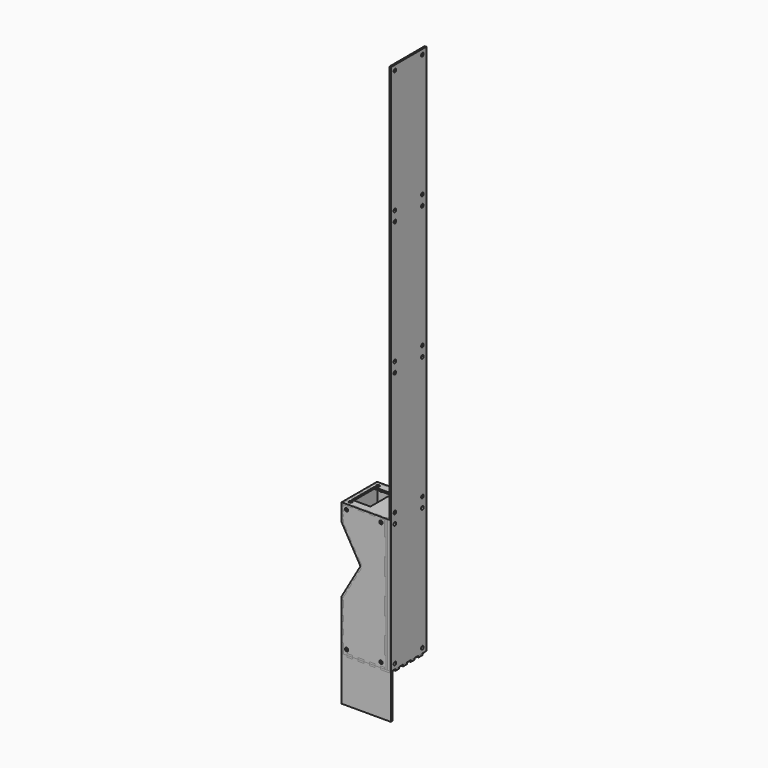
from build123d import *

# Parameters (mm, degrees)
F5_W      = 7
F5_H      = 3
F5_W_2    = 10
F5_W_3    = 3
F5_H_2    = 5.9052353799
F5_H_3    = 8.75
F5_R      = 3
F5_W_4    = 33.25
F5_H_4    = 50
F5_H_5    = 6.8447646201
F27_DEPTH = 3
F7_R      = 3
F7_W      = 3
F7_H      = 30
F7_H_2    = 31.25
F7_H_3    = 22.5
F28_DEPTH = 3
F3_R      = 3
F29_DEPTH = 3
F9_W      = 7
F9_H      = 3
F9_W_2    = 10
F9_R      = 3
F9_W_3    = 3
F9_H_2    = 15.5947646201
F9_H_3    = 8.75
F9_H_4    = 5.9052353799
F30_DEPTH = 3
F11_R     = 3
F31_DEPTH = 3
F32_DEPTH = 3
F33_DEPTH = 3
F34_DEPTH = 3
F35_DEPTH = 3
F36_DEPTH = 3
F37_DEPTH = 3
F38_DEPTH = 3
F39_DEPTH = 3
F40_DEPTH = 3
F19_R     = 25
F41_DEPTH = 3
F42_DEPTH = 3
F21_R     = 3
F43_DEPTH = 3
F22_W     = 80
F22_H     = 240
F22_R     = 3
F22_W_2   = 2
F22_H_2   = 144
F22_W_3   = 12
F44_DEPTH = 3
F24_W     = 80
F24_H     = 240
F24_R     = 3
F45_DEPTH = 3
F26_R     = 3
F26_W     = 3
F26_H     = 2
F26_W_2   = 33.25
F26_H_2   = 50
F46_DEPTH = 3
F47_DEPTH = 3
F25_W     = 7
F25_H     = 3
F25_W_2   = 3
F25_H_2   = 8.75
F25_W_3   = 10
F25_H_3   = 5.9052353799
F48_DEPTH = 3
F25_H_4   = 6.8447646201
F49_DEPTH = 3


# Not quite as in the source:
# - a feature names something its author has since deleted; it is built from what else it names


with BuildPart() as f27:
    # F5 (on line) → F27 (new body)
    with BuildSketch(Plane.XY.offset(240)):
        with Locations((-73.5, 78.5)):
            Rectangle(F5_W, F5_H)
        with Locations((-55, 78.5)):
            Rectangle(F5_W_2, F5_H)
        with Locations((-35, 78.5)):
            Rectangle(F5_W_2, F5_H)
        with Locations((-15, 78.5)):
            Rectangle(F5_W_2, F5_H)
        with Locations((-1.5, 78.5)):
            Rectangle(F5_W_3, F5_H)
        with Locations((-1.5, 74.04738231)):
            Rectangle(F5_W_3, F5_H_2)
        with Locations((-1.5, 57.9697646201)):
            Rectangle(F5_W_3, F5_H_3)
        with Locations((-1.5, 40.4697646201)):
            Rectangle(F5_W_3, F5_H_3)
        with Locations((-1.5, 22.9697646201)):
            Rectangle(F5_W_3, F5_H_3)
        with Locations((-25, 1.5)):
            Rectangle(F5_W_2, F5_H)
        with Locations((-45, 1.5)):
            Rectangle(F5_W_2, F5_H)
        with Locations((-65, 1.5)):
            Rectangle(F5_W_2, F5_H)
        with Locations((-78.5, 66.7197646201)):
            Rectangle(F5_W_3, F5_H_3)
        with Locations((-78.5, 49.2197646201)):
            Rectangle(F5_W_3, F5_H_3)
        with Locations((-78.5, 31.7197646201)):
            Rectangle(F5_W_3, F5_H_3)
        with Locations((-78.5, 14.2197646201)):
            Rectangle(F5_W_3, F5_H_3)
        Polygon((-77, 9.8447646201), (-77, 3), (-70, 3), (-60, 3), (-50, 3), (-40, 3), (-30, 3), (-20, 3), (-10, 3), (-3, 3), (-3, 9.8447646201), (-3, 18.5947646201), (-3, 27.3447646201), (-3, 36.0947646201), (-3, 44.8447646201), (-3, 53.5947646201), (-3, 62.3447646201), (-3, 71.0947646201), (-3, 77), (-10, 77), (-20, 77), (-30, 77), (-40, 77), (-50, 77), (-60, 77), (-70, 77), (-77, 77), (-77, 71.0947646201), (-77, 62.3447646201), (-77, 53.5947646201), (-77, 44.8447646201), (-77, 36.0947646201), (-77, 27.3447646201), (-77, 18.5947646201), align=None)
        with Locations((-71, 9)):
            Circle(F5_R, mode=Mode.SUBTRACT)
        with Locations((-56.625, 40)):
            Rectangle(F5_W_4, F5_H_4, mode=Mode.SUBTRACT)
        with Locations((-71, 71)):
            Circle(F5_R, mode=Mode.SUBTRACT)
        with Locations((-9, 40)):
            Circle(F5_R, mode=Mode.SUBTRACT)
        with Locations((-1.5, 6.42238231)):
            Rectangle(F5_W_3, F5_H_5)
        with Locations((-6.5, 1.5)):
            Rectangle(F5_W, F5_H)
        with Locations((-78.5, 1.5)):
            Rectangle(F5_W_3, F5_H)
        with Locations((-73.5, 1.5)):
            Rectangle(F5_W, F5_H)
    extrude(amount=-F27_DEPTH)


with BuildPart() as f28:
    # F7 (on line) → F28 (new body)
    with BuildSketch(Plane.YZ):
        Polygon((3, 22.5), (3, 0), (77, 0), (77, 22.5), (77, 53.75), (77, 85), (77, 116.25), (77, 147.5), (77, 178.75), (77, 210), (77, 240), (3, 240), (3, 210), (3, 178.75), (3, 147.5), (3, 116.25), (3, 85), (3, 53.75), align=None)
        with Locations((9, 9)):
            Circle(F7_R, mode=Mode.SUBTRACT)
        with Locations((71, 9)):
            Circle(F7_R, mode=Mode.SUBTRACT)
        with Locations((9, 231)):
            Circle(F7_R, mode=Mode.SUBTRACT)
        with Locations((71, 231)):
            Circle(F7_R, mode=Mode.SUBTRACT)
        with Locations((1.5, 225)):
            Rectangle(F7_W, F7_H)
        with Locations((1.5, 163.125)):
            Rectangle(F7_W, F7_H_2)
        with Locations((1.5, 100.625)):
            Rectangle(F7_W, F7_H_2)
        with Locations((1.5, 38.125)):
            Rectangle(F7_W, F7_H_2)
        with Locations((78.5, 11.25)):
            Rectangle(F7_W, F7_H_3)
        with Locations((78.5, 69.375)):
            Rectangle(F7_W, F7_H_2)
        with Locations((78.5, 131.875)):
            Rectangle(F7_W, F7_H_2)
        with Locations((78.5, 194.375)):
            Rectangle(F7_W, F7_H_2)
    extrude(amount=-F28_DEPTH)


with BuildPart() as f29:
    # F3 (on Front) → F29 (new body)
    with BuildSketch(Plane.XZ):
        Polygon((0, 240), (-80, 240), (-80, 208.334591186), (-46, 149.4448637287), (-80, 90.5551362713), (-80, 0), (0, 0), align=None)
        with Locations((-71, 9)):
            Circle(F3_R, mode=Mode.SUBTRACT)
        with Locations((-9, 9)):
            Circle(F3_R, mode=Mode.SUBTRACT)
        with Locations((-71, 231)):
            Circle(F3_R, mode=Mode.SUBTRACT)
        with Locations((-9, 231)):
            Circle(F3_R, mode=Mode.SUBTRACT)
    extrude(amount=-F29_DEPTH)


with BuildPart() as f30:
    # F9 (on line) → F30 (new body)
    with BuildSketch(Plane.XY):
        with Locations((-6.5, 1.5)):
            Rectangle(F9_W, F9_H)
        with Locations((-25, 1.5)):
            Rectangle(F9_W_2, F9_H)
        with Locations((-45, 1.5)):
            Rectangle(F9_W_2, F9_H)
        with Locations((-65, 1.5)):
            Rectangle(F9_W_2, F9_H)
        Polygon((-77, 18.5947646201), (-77, 3), (-70, 3), (-60, 3), (-50, 3), (-40, 3), (-30, 3), (-20, 3), (-10, 3), (-3, 3), (-3, 18.5947646201), (-3, 27.3447646201), (-3, 36.0947646201), (-3, 44.8447646201), (-3, 53.5947646201), (-3, 62.3447646201), (-3, 71.0947646201), (-3, 77), (-10, 77), (-20, 77), (-30, 77), (-40, 77), (-50, 77), (-60, 77), (-70, 77), (-77, 77), (-77, 71.0947646201), (-77, 62.3447646201), (-77, 53.5947646201), (-77, 44.8447646201), (-77, 36.0947646201), (-77, 27.3447646201), align=None)
        with Locations((-71, 9)):
            Circle(F9_R, mode=Mode.SUBTRACT)
        with BuildLine():
            ThreePointArc((-67.25, 32), (-70.25, 29), (-73.25, 32))
            ThreePointArc((-73.25, 32), (-70.25, 35), (-67.25, 32))
        make_face(mode=Mode.SUBTRACT)
        with Locations((-62.25, 36)):
            Circle(F9_R, mode=Mode.SUBTRACT)
        with BuildLine():
            ThreePointArc((-67.25, 40), (-70.25, 37), (-73.25, 40))
            ThreePointArc((-73.25, 40), (-70.25, 43), (-67.25, 40))
        make_face(mode=Mode.SUBTRACT)
        with BuildLine():
            ThreePointArc((-67.25, 48), (-70.25, 45), (-73.25, 48))
            ThreePointArc((-73.25, 48), (-70.25, 51), (-67.25, 48))
        make_face(mode=Mode.SUBTRACT)
        with Locations((-62.25, 44)):
            Circle(F9_R, mode=Mode.SUBTRACT)
        with Locations((-54.25, 40)):
            Circle(F9_R, mode=Mode.SUBTRACT)
        with Locations((-71, 71)):
            Circle(F9_R, mode=Mode.SUBTRACT)
        with BuildLine():
            ThreePointArc((-6.75, 41.9843134833), (-6.1937569599, 41.0606601718), (-6, 40))
            ThreePointArc((-6, 40), (-11.8062430401, 38.9393398282), (-6.75, 41.9843134833))
        make_face(mode=Mode.SUBTRACT)
        with Locations((-78.5, 10.79738231)):
            Rectangle(F9_W_3, F9_H_2)
        with Locations((-78.5, 31.7197646201)):
            Rectangle(F9_W_3, F9_H_3)
        with Locations((-1.5, 22.9697646201)):
            Rectangle(F9_W_3, F9_H_3)
        with Locations((-1.5, 40.4697646201)):
            Rectangle(F9_W_3, F9_H_3)
        with Locations((-1.5, 57.9697646201)):
            Rectangle(F9_W_3, F9_H_3)
        with Locations((-1.5, 74.04738231)):
            Rectangle(F9_W_3, F9_H_4)
        with Locations((-1.5, 78.5)):
            Rectangle(F9_W_3, F9_H)
        with Locations((-15, 78.5)):
            Rectangle(F9_W_2, F9_H)
        with Locations((-35, 78.5)):
            Rectangle(F9_W_2, F9_H)
        with Locations((-55, 78.5)):
            Rectangle(F9_W_2, F9_H)
        with Locations((-73.5, 78.5)):
            Rectangle(F9_W, F9_H)
        with Locations((-78.5, 66.7197646201)):
            Rectangle(F9_W_3, F9_H_3)
        with Locations((-78.5, 49.2197646201)):
            Rectangle(F9_W_3, F9_H_3)
        with Locations((-78.5, 1.5)):
            Rectangle(F9_W_3, F9_H)
    extrude(amount=F30_DEPTH)


with BuildPart() as f31:
    # F11 (on line) → F31 (new body)
    with BuildSketch(Plane(origin=(0, 80, 0), x_dir=(-1, 0, 0), z_dir=(0, 1, 0))):
        Polygon((46, 149.4448637287), (80, 208.334591186), (80, 240), (0, 240), (0, 0), (80, 0), (80, 90.5551362713), align=None)
        with Locations((9, 9)):
            Circle(F11_R, mode=Mode.SUBTRACT)
        with Locations((71, 9)):
            Circle(F11_R, mode=Mode.SUBTRACT)
        with Locations((9, 231)):
            Circle(F11_R, mode=Mode.SUBTRACT)
        with Locations((71, 231)):
            Circle(F11_R, mode=Mode.SUBTRACT)
    extrude(amount=-F31_DEPTH)


with BuildPart() as f32:
    # F13 (on line) → F32 (new body)
    with BuildSketch(Plane.YZ.offset(-80)):
        Polygon((0, 213.8509433895), (0, 208.334591186), (80, 208.334591186), (80, 213.8509433895), (77, 213.8509433895), (77, 216.2509433895), (77, 218.6509433895), (80, 218.6509433895), (80, 221.767295593), (77, 221.767295593), (77, 224.167295593), (77, 226.567295593), (80, 226.567295593), (80, 229.6836477965), (77, 229.6836477965), (77, 232.0836477965), (77, 234.4836477965), (80, 234.4836477965), (80, 240), (0, 240), (0, 234.4836477965), (3, 234.4836477965), (3, 232.0836477965), (3, 229.6836477965), (0, 229.6836477965), (0, 226.567295593), (3, 226.567295593), (3, 224.167295593), (3, 221.767295593), (0, 221.767295593), (0, 218.6509433895), (3, 218.6509433895), (3, 216.2509433895), (3, 213.8509433895), align=None)
    extrude(amount=F32_DEPTH)


with BuildPart() as f33:
    # F15 (on line) → F33 (new body)
    with BuildSketch(Plane.YZ.offset(-80)):
        Polygon((77.0001318272, 51.2494443715), (80, 51.2775681357), (80, 60.7913522035), (77.0001318272, 60.7913522035), (77.0001318272, 66.7913522035), (77.0001318272, 72.7913522035), (80, 72.7913522035), (80, 85.3051362713), (77.0001318272, 85.3051362713), (77.0001318272, 89.0551362713), (2.9998681728, 89.0551362713), (2.9998681728, 85.3051362713), (0, 85.3051362713), (0, 72.7913522035), (2.9998681728, 72.7913522035), (2.9998681728, 66.7913522035), (2.9998681728, 60.7913522035), (0, 60.7913522035), (0, 51.2775681357), (2.9998681728, 51.2494443715), (2.9998681728, 45.2494443715), (2.8873780596, 39.2504989664), (0, 39.2775681357), (0, 29.7610567958), (2.7084830109, 29.7102682755), (2.5959928978, 23.7113228703), (2.4835027846, 17.7123774651), (0, 17.7589472354), (0, 0), (80, 0), (80, 17.7589472354), (77.5164972154, 17.7123774651), (77.4040071022, 23.7113228703), (77.2915169891, 29.7102682755), (80, 29.7610567958), (80, 39.2775681357), (77.1126219404, 39.2504989664), (77.0001318272, 45.2494443715), align=None)
    extrude(amount=F33_DEPTH)


with BuildPart() as f34_tool:
    # F5 (on line) → F34 (new body)
    with BuildSketch(Plane.XY.offset(240)):
        with Locations((-1.5, 22.9697646201)):
            Rectangle(F5_W_3, F5_H_3)
        with Locations((-1.5, 40.4697646201)):
            Rectangle(F5_W_3, F5_H_3)
        with Locations((-1.5, 57.9697646201)):
            Rectangle(F5_W_3, F5_H_3)
        with Locations((-1.5, 74.04738231)):
            Rectangle(F5_W_3, F5_H_2)
        with Locations((-1.5, 78.5)):
            Rectangle(F5_W_3, F5_H)
        with Locations((-15, 78.5)):
            Rectangle(F5_W_2, F5_H)
        with Locations((-35, 78.5)):
            Rectangle(F5_W_2, F5_H)
        with Locations((-55, 78.5)):
            Rectangle(F5_W_2, F5_H)
        with Locations((-73.5, 78.5)):
            Rectangle(F5_W, F5_H)
        with Locations((-78.5, 66.7197646201)):
            Rectangle(F5_W_3, F5_H_3)
        with Locations((-78.5, 49.2197646201)):
            Rectangle(F5_W_3, F5_H_3)
        with Locations((-78.5, 31.7197646201)):
            Rectangle(F5_W_3, F5_H_3)
        with Locations((-78.5, 14.2197646201)):
            Rectangle(F5_W_3, F5_H_3)
        with Locations((-78.5, 1.5)):
            Rectangle(F5_W_3, F5_H)
        with Locations((-65, 1.5)):
            Rectangle(F5_W_2, F5_H)
        with Locations((-45, 1.5)):
            Rectangle(F5_W_2, F5_H)
        with Locations((-25, 1.5)):
            Rectangle(F5_W_2, F5_H)
        with Locations((-6.5, 1.5)):
            Rectangle(F5_W, F5_H)
        with Locations((-73.5, 1.5)):
            Rectangle(F5_W, F5_H)
        with Locations((-1.5, 6.42238231)):
            Rectangle(F5_W_3, F5_H_5)
    extrude(amount=-F34_DEPTH)


with BuildPart() as f28_1:
    add(f28.part)

    # F34: cut by f34_tool
    add(f34_tool.part, mode=Mode.SUBTRACT)


with BuildPart() as f29_1:
    add(f29.part)

    # F34: cut by f34_tool
    add(f34_tool.part, mode=Mode.SUBTRACT)


with BuildPart() as f31_1:
    add(f31.part)

    # F34: cut by f34_tool
    add(f34_tool.part, mode=Mode.SUBTRACT)


with BuildPart() as f32_1:
    add(f32.part)

    # F34: cut by f34_tool
    add(f34_tool.part, mode=Mode.SUBTRACT)


with BuildPart() as f35_tool:
    # F7 (on line) → F35 (new body)
    with BuildSketch(Plane.YZ):
        with Locations((1.5, 225)):
            Rectangle(F7_W, F7_H)
        with Locations((78.5, 194.375)):
            Rectangle(F7_W, F7_H_2)
        with Locations((1.5, 163.125)):
            Rectangle(F7_W, F7_H_2)
        with Locations((78.5, 131.875)):
            Rectangle(F7_W, F7_H_2)
        with Locations((1.5, 100.625)):
            Rectangle(F7_W, F7_H_2)
        with Locations((78.5, 69.375)):
            Rectangle(F7_W, F7_H_2)
        with Locations((1.5, 38.125)):
            Rectangle(F7_W, F7_H_2)
        with Locations((78.5, 11.25)):
            Rectangle(F7_W, F7_H_3)
    extrude(amount=-F35_DEPTH)


with BuildPart() as f29_2:
    add(f29_1.part)

    # F35: cut by f35_tool
    add(f35_tool.part, mode=Mode.SUBTRACT)


with BuildPart() as f31_2:
    add(f31_1.part)

    # F35: cut by f35_tool
    add(f35_tool.part, mode=Mode.SUBTRACT)


with BuildPart() as f36_tool:
    # F13 (on line) → F36 (new body)
    with BuildSketch(Plane.YZ.offset(-80)):
        Polygon((0, 213.8509433895), (0, 208.334591186), (80, 208.334591186), (80, 213.8509433895), (77, 213.8509433895), (77, 216.2509433895), (77, 218.6509433895), (80, 218.6509433895), (80, 221.767295593), (77, 221.767295593), (77, 224.167295593), (77, 226.567295593), (80, 226.567295593), (80, 229.6836477965), (77, 229.6836477965), (77, 232.0836477965), (77, 234.4836477965), (80, 234.4836477965), (80, 240), (0, 240), (0, 234.4836477965), (3, 234.4836477965), (3, 232.0836477965), (3, 229.6836477965), (0, 229.6836477965), (0, 226.567295593), (3, 226.567295593), (3, 224.167295593), (3, 221.767295593), (0, 221.767295593), (0, 218.6509433895), (3, 218.6509433895), (3, 216.2509433895), (3, 213.8509433895), align=None)
    extrude(amount=F36_DEPTH)


with BuildPart() as f29_3:
    add(f29_2.part)

    # F36: cut by f36_tool
    add(f36_tool.part, mode=Mode.SUBTRACT)


with BuildPart() as f31_3:
    add(f31_2.part)

    # F36: cut by f36_tool
    add(f36_tool.part, mode=Mode.SUBTRACT)


with BuildPart() as f37_tool:
    # F15 (on line) → F37 (new body)
    with BuildSketch(Plane.YZ.offset(-80)):
        Polygon((77.0001318272, 51.2494443715), (80, 51.2775681357), (80, 60.7913522035), (77.0001318272, 60.7913522035), (77.0001318272, 66.7913522035), (77.0001318272, 72.7913522035), (80, 72.7913522035), (80, 85.3051362713), (77.0001318272, 85.3051362713), (77.0001318272, 89.0551362713), (2.9998681728, 89.0551362713), (2.9998681728, 85.3051362713), (0, 85.3051362713), (0, 72.7913522035), (2.9998681728, 72.7913522035), (2.9998681728, 66.7913522035), (2.9998681728, 60.7913522035), (0, 60.7913522035), (0, 51.2775681357), (2.9998681728, 51.2494443715), (2.9998681728, 45.2494443715), (2.8873780596, 39.2504989664), (0, 39.2775681357), (0, 29.7610567958), (2.7084830109, 29.7102682755), (2.5959928978, 23.7113228703), (2.4835027846, 17.7123774651), (0, 17.7589472354), (0, 0), (80, 0), (80, 17.7589472354), (77.5164972154, 17.7123774651), (77.4040071022, 23.7113228703), (77.2915169891, 29.7102682755), (80, 29.7610567958), (80, 39.2775681357), (77.1126219404, 39.2504989664), (77.0001318272, 45.2494443715), align=None)
    extrude(amount=F37_DEPTH)


with BuildPart() as f29_4:
    add(f29_3.part)

    # F37: cut by f37_tool
    add(f37_tool.part, mode=Mode.SUBTRACT)


with BuildPart() as f31_4:
    add(f31_3.part)

    # F37: cut by f37_tool
    add(f37_tool.part, mode=Mode.SUBTRACT)


with BuildPart() as f38_tool:
    # F9 (on line) → F38 (new body)
    with BuildSketch(Plane.XY):
        with Locations((-73.5, 78.5)):
            Rectangle(F9_W, F9_H)
        with Locations((-78.5, 66.7197646201)):
            Rectangle(F9_W_3, F9_H_3)
        with Locations((-55, 78.5)):
            Rectangle(F9_W_2, F9_H)
        with Locations((-35, 78.5)):
            Rectangle(F9_W_2, F9_H)
        with Locations((-15, 78.5)):
            Rectangle(F9_W_2, F9_H)
        with Locations((-1.5, 78.5)):
            Rectangle(F9_W_3, F9_H)
        with Locations((-1.5, 74.04738231)):
            Rectangle(F9_W_3, F9_H_4)
        with Locations((-1.5, 57.9697646201)):
            Rectangle(F9_W_3, F9_H_3)
        with Locations((-1.5, 40.4697646201)):
            Rectangle(F9_W_3, F9_H_3)
        with Locations((-1.5, 22.9697646201)):
            Rectangle(F9_W_3, F9_H_3)
        with Locations((-6.5, 1.5)):
            Rectangle(F9_W, F9_H)
        with Locations((-25, 1.5)):
            Rectangle(F9_W_2, F9_H)
        with Locations((-45, 1.5)):
            Rectangle(F9_W_2, F9_H)
        with Locations((-65, 1.5)):
            Rectangle(F9_W_2, F9_H)
        with Locations((-78.5, 1.5)):
            Rectangle(F9_W_3, F9_H)
        with Locations((-78.5, 10.79738231)):
            Rectangle(F9_W_3, F9_H_2)
        with Locations((-78.5, 31.7197646201)):
            Rectangle(F9_W_3, F9_H_3)
        with Locations((-78.5, 49.2197646201)):
            Rectangle(F9_W_3, F9_H_3)
    extrude(amount=F38_DEPTH)


with BuildPart() as f28_2:
    add(f28_1.part)

    # F38: cut by f38_tool
    add(f38_tool.part, mode=Mode.SUBTRACT)


with BuildPart() as f29_5:
    add(f29_4.part)

    # F38: cut by f38_tool
    add(f38_tool.part, mode=Mode.SUBTRACT)


with BuildPart() as f31_5:
    add(f31_4.part)

    # F38: cut by f38_tool
    add(f38_tool.part, mode=Mode.SUBTRACT)


with BuildPart() as f33_1:
    add(f33.part)

    # F38: cut by f38_tool
    add(f38_tool.part, mode=Mode.SUBTRACT)


with BuildPart() as f39:
    # F17 (on line) → F39 (new body)
    with BuildSketch(Plane(origin=(30.2115242271, 0, 17.4426316451), x_dir=(0, 1, 0), z_dir=(0.8660254038, 0, 0.5))):
        Polygon((0, 166.4230484541), (0, 153.2890738579), (80, 153.2890738579), (80, 166.4230484541), (77, 166.4230484541), (77, 170.1730484541), (77, 173.9230484541), (80, 173.9230484541), (80, 182.6730484541), (77, 182.6730484541), (77, 186.4230484541), (77, 190.1730484541), (80, 190.1730484541), (80, 198.9230484541), (77, 198.9230484541), (77, 202.6730484541), (77, 206.4230484541), (80, 206.4230484541), (80, 215.1730484541), (77, 215.1730484541), (77, 218.9230484541), (3, 218.9230484541), (3, 215.1730484541), (0, 215.1730484541), (0, 206.4230484541), (3, 206.4230484541), (3, 202.6730484541), (3, 198.9230484541), (0, 198.9230484541), (0, 190.1730484541), (3, 190.1730484541), (3, 186.4230484541), (3, 182.6730484541), (0, 182.6730484541), (0, 173.9230484541), (3, 173.9230484541), (3, 170.1730484541), (3, 166.4230484541), align=None)
    extrude(amount=F39_DEPTH)


with BuildPart() as f40_tool:
    # F17 (on line) → F40 (new body)
    with BuildSketch(Plane(origin=(30.2115242271, 0, 17.4426316451), x_dir=(0, 1, 0), z_dir=(0.8660254038, 0, 0.5))):
        Polygon((0, 166.4230484541), (0, 153.2890738579), (80, 153.2890738579), (80, 166.4230484541), (77, 166.4230484541), (77, 170.1730484541), (77, 173.9230484541), (80, 173.9230484541), (80, 182.6730484541), (77, 182.6730484541), (77, 186.4230484541), (77, 190.1730484541), (80, 190.1730484541), (80, 198.9230484541), (77, 198.9230484541), (77, 202.6730484541), (77, 206.4230484541), (80, 206.4230484541), (80, 215.1730484541), (77, 215.1730484541), (77, 218.9230484541), (3, 218.9230484541), (3, 215.1730484541), (0, 215.1730484541), (0, 206.4230484541), (3, 206.4230484541), (3, 202.6730484541), (3, 198.9230484541), (0, 198.9230484541), (0, 190.1730484541), (3, 190.1730484541), (3, 186.4230484541), (3, 182.6730484541), (0, 182.6730484541), (0, 173.9230484541), (3, 173.9230484541), (3, 170.1730484541), (3, 166.4230484541), align=None)
    extrude(amount=F40_DEPTH)


with BuildPart() as f29_6:
    add(f29_5.part)

    # F40: cut by f40_tool
    add(f40_tool.part, mode=Mode.SUBTRACT)


with BuildPart() as f31_6:
    add(f31_5.part)

    # F40: cut by f40_tool
    add(f40_tool.part, mode=Mode.SUBTRACT)


with BuildPart() as f41:
    # F19 (on line) → F41 (new body)
    with BuildSketch(Plane(origin=(-99.2115242271, 0, 57.2798002192), x_dir=(0, 1, 0), z_dir=(0.8660254038, 0, -0.5))):
        Polygon((0, 52.106061156), (0, 38.4230484541), (80, 38.4230484541), (80, 52.106061156), (77, 52.106061156), (77, 55.856061156), (77, 59.606061156), (80, 59.606061156), (80, 69.5390738579), (77, 69.5390738579), (77, 73.2890738579), (77, 77.0390738579), (80, 77.0390738579), (80, 86.9720865598), (77, 86.9720865598), (77, 90.7220865598), (77, 94.4720865598), (80, 94.4720865598), (80, 104.4050992617), (77, 104.4050992617), (77, 108.1550992617), (3, 108.1550992617), (3, 104.4050992617), (0, 104.4050992617), (0, 94.4720865598), (3, 94.4720865598), (3, 90.7220865598), (3, 86.9720865598), (0, 86.9720865598), (0, 77.0390738579), (3, 77.0390738579), (3, 73.2890738579), (3, 69.5390738579), (0, 69.5390738579), (0, 59.606061156), (3, 59.606061156), (3, 55.856061156), (3, 52.106061156), align=None)
        with Locations((40, 73.2890738579)):
            Circle(F19_R, mode=Mode.SUBTRACT)
    extrude(amount=F41_DEPTH)


with BuildPart() as f42_tool:
    # F19 (on line) → F42 (new body)
    with BuildSketch(Plane(origin=(-99.2115242271, 0, 57.2798002192), x_dir=(0, 1, 0), z_dir=(0.8660254038, 0, -0.5))):
        Polygon((0, 52.106061156), (0, 38.4230484541), (80, 38.4230484541), (80, 52.106061156), (77, 52.106061156), (77, 55.856061156), (77, 59.606061156), (80, 59.606061156), (80, 69.5390738579), (77, 69.5390738579), (77, 73.2890738579), (77, 77.0390738579), (80, 77.0390738579), (80, 86.9720865598), (77, 86.9720865598), (77, 90.7220865598), (77, 94.4720865598), (80, 94.4720865598), (80, 104.4050992617), (77, 104.4050992617), (77, 108.1550992617), (3, 108.1550992617), (3, 104.4050992617), (0, 104.4050992617), (0, 94.4720865598), (3, 94.4720865598), (3, 90.7220865598), (3, 86.9720865598), (0, 86.9720865598), (0, 77.0390738579), (3, 77.0390738579), (3, 73.2890738579), (3, 69.5390738579), (0, 69.5390738579), (0, 59.606061156), (3, 59.606061156), (3, 55.856061156), (3, 52.106061156), align=None)
        with Locations((40, 73.2890738579)):
            Circle(F19_R, mode=Mode.SUBTRACT)
    extrude(amount=F42_DEPTH)


with BuildPart() as f29_7:
    add(f29_6.part)

    # F42: cut by f42_tool
    add(f42_tool.part, mode=Mode.SUBTRACT)


with BuildPart() as f31_7:
    add(f31_6.part)

    # F42: cut by f42_tool
    add(f42_tool.part, mode=Mode.SUBTRACT)


with BuildPart() as f43:
    # F21 (on offset) → F43 (new body)
    with BuildSketch(Plane.YZ.offset(3)):
        Polygon((0, 240), (0, 0), (18, 0), (18, 80), (20, 80), (20, 0), (22, 0), (22, 80), (24, 80), (24, 0), (26, 0), (26, 80), (28, 80), (28, 0), (30, 0), (30, 80), (32, 80), (32, 0), (34, 0), (34, 80), (36, 80), (36, 0), (38, 0), (38, 80), (40, 80), (40, 0), (54, 0), (54, 80), (66, 80), (66, 0), (80, 0), (80, 240), (66, 240), (66, 160), (54, 160), (54, 240), (40, 240), (40, 160), (38, 160), (38, 240), (36, 240), (36, 160), (34, 160), (34, 240), (32, 240), (32, 160), (30, 160), (30, 240), (28, 240), (28, 160), (26, 160), (26, 240), (24, 240), (24, 160), (22, 160), (22, 240), (20, 240), (20, 160), (18, 160), (18, 240), align=None)
        with Locations((9, 9)):
            Circle(F21_R, mode=Mode.SUBTRACT)
        with Locations((71, 9)):
            Circle(F21_R, mode=Mode.SUBTRACT)
        with Locations((9, 231)):
            Circle(F21_R, mode=Mode.SUBTRACT)
        with Locations((71, 231)):
            Circle(F21_R, mode=Mode.SUBTRACT)
    extrude(amount=-F43_DEPTH)


with BuildPart() as f44:
    # F22 (on offset) → F44 (new body)
    with BuildSketch(Plane.YZ.offset(3)):
        with Locations((40, 120)):
            Rectangle(F22_W, F22_H)
        with Locations((9, 9)):
            Circle(F22_R, mode=Mode.SUBTRACT)
        with Locations((71, 9)):
            Circle(F22_R, mode=Mode.SUBTRACT)
        with Locations((19, 120)):
            Rectangle(F22_W_2, F22_H_2, mode=Mode.SUBTRACT)
        with Locations((23, 120)):
            Rectangle(F22_W_2, F22_H_2, mode=Mode.SUBTRACT)
        with Locations((27, 120)):
            Rectangle(F22_W_2, F22_H_2, mode=Mode.SUBTRACT)
        with Locations((31, 120)):
            Rectangle(F22_W_2, F22_H_2, mode=Mode.SUBTRACT)
        with Locations((35, 120)):
            Rectangle(F22_W_2, F22_H_2, mode=Mode.SUBTRACT)
        with Locations((39, 120)):
            Rectangle(F22_W_2, F22_H_2, mode=Mode.SUBTRACT)
        with Locations((9, 231)):
            Circle(F22_R, mode=Mode.SUBTRACT)
        with Locations((60, 120)):
            Rectangle(F22_W_3, F22_H_2, mode=Mode.SUBTRACT)
        with Locations((71, 231)):
            Circle(F22_R, mode=Mode.SUBTRACT)
    extrude(amount=F44_DEPTH)


with BuildPart() as f45:
    # F24 (on offset) → F45 (new body)
    with BuildSketch(Plane.YZ.offset(9)):
        with Locations((40, 120)):
            Rectangle(F24_W, F24_H)
        with Locations((9, 9)):
            Circle(F24_R, mode=Mode.SUBTRACT)
        with Locations((9, 231)):
            Circle(F24_R, mode=Mode.SUBTRACT)
        with Locations((71, 9)):
            Circle(F24_R, mode=Mode.SUBTRACT)
        with Locations((71, 231)):
            Circle(F24_R, mode=Mode.SUBTRACT)
        with Locations((40, 360)):
            Rectangle(F24_W, F24_H)
        with Locations((9, 249)):
            Circle(F24_R, mode=Mode.SUBTRACT)
        with Locations((9, 471)):
            Circle(F24_R, mode=Mode.SUBTRACT)
        with Locations((71, 249)):
            Circle(F24_R, mode=Mode.SUBTRACT)
        with Locations((71, 471)):
            Circle(F24_R, mode=Mode.SUBTRACT)
        with Locations((40, 600)):
            Rectangle(F24_W, F24_H)
        with Locations((9, 489)):
            Circle(F24_R, mode=Mode.SUBTRACT)
        with Locations((9, 711)):
            Circle(F24_R, mode=Mode.SUBTRACT)
        with Locations((71, 489)):
            Circle(F24_R, mode=Mode.SUBTRACT)
        with Locations((71, 711)):
            Circle(F24_R, mode=Mode.SUBTRACT)
        with Locations((40, 840)):
            Rectangle(F24_W, F24_H)
        with Locations((9, 729)):
            Circle(F24_R, mode=Mode.SUBTRACT)
        with Locations((9, 951)):
            Circle(F24_R, mode=Mode.SUBTRACT)
        with Locations((71, 729)):
            Circle(F24_R, mode=Mode.SUBTRACT)
        with Locations((71, 951)):
            Circle(F24_R, mode=Mode.SUBTRACT)
    extrude(amount=-F45_DEPTH)


with BuildPart() as f46:
    # F26 (on line) → F46 (new body)
    with BuildSketch(Plane.XY):
        Polygon((0, 80), (-80, 80), (-80, 0), (0, 0), (9, 0), (9, 80), align=None)
        with Locations((-71, 9)):
            Circle(F26_R, mode=Mode.SUBTRACT)
        with Locations((1.5, 19)):
            Rectangle(F26_W, F26_H, mode=Mode.SUBTRACT)
        with Locations((1.5, 23)):
            Rectangle(F26_W, F26_H, mode=Mode.SUBTRACT)
        with Locations((1.5, 27)):
            Rectangle(F26_W, F26_H, mode=Mode.SUBTRACT)
        with Locations((1.5, 31)):
            Rectangle(F26_W, F26_H, mode=Mode.SUBTRACT)
        with Locations((1.5, 35)):
            Rectangle(F26_W, F26_H, mode=Mode.SUBTRACT)
        with Locations((1.5, 39)):
            Rectangle(F26_W, F26_H, mode=Mode.SUBTRACT)
        with Locations((-56.625, 40)):
            Rectangle(F26_W_2, F26_H_2, mode=Mode.SUBTRACT)
        with Locations((-71, 71)):
            Circle(F26_R, mode=Mode.SUBTRACT)
        with Locations((-9, 40)):
            Circle(F26_R, mode=Mode.SUBTRACT)
    extrude(amount=-F46_DEPTH)

    # F25 (on line) → F48 (cut)
    with BuildSketch(Plane.XY):
        with Locations((-73.5, 78.5)):
            Rectangle(F25_W, F25_H)
        with Locations((-78.5, 66.7197646201)):
            Rectangle(F25_W_2, F25_H_2)
        with Locations((-78.5, 49.2197646201)):
            Rectangle(F25_W_2, F25_H_2)
        with Locations((-78.5, 31.7197646201)):
            Rectangle(F25_W_2, F25_H_2)
        with Locations((-78.5, 14.2197646201)):
            Rectangle(F25_W_2, F25_H_2)
        with Locations((-78.5, 1.5)):
            Rectangle(F25_W_2, F25_H)
        with Locations((-73.5, 1.5)):
            Rectangle(F25_W, F25_H)
        with Locations((-55, 1.5)):
            Rectangle(F25_W_3, F25_H)
        Polygon((-30.25, 3), (-33.25, 3), (-40, 3), (-40, 0), (-30, 0), (-30, 3), align=None)
        with Locations((-15, 1.5)):
            Rectangle(F25_W_3, F25_H)
        with Locations((7.5, 1.5)):
            Rectangle(F25_W_2, F25_H)
        Polygon((6, 9.8447646201), (6, 3), (9, 3), (9, 9.7607485838), align=None)
        with Locations((7.5, 22.9697646201)):
            Rectangle(F25_W_2, F25_H_2)
        with Locations((7.5, 40.4697646201)):
            Rectangle(F25_W_2, F25_H_2)
        with Locations((7.5, 57.9697646201)):
            Rectangle(F25_W_2, F25_H_2)
        with Locations((7.5, 74.04738231)):
            Rectangle(F25_W_2, F25_H_3)
        with Locations((7.5, 78.5)):
            Rectangle(F25_W_2, F25_H)
        with Locations((-15, 78.5)):
            Rectangle(F25_W_3, F25_H)
        Polygon((-30, 80), (-40, 80), (-40, 77), (-33.25, 77), (-30.25, 77), (-30, 77), align=None)
        with Locations((-55, 78.5)):
            Rectangle(F25_W_3, F25_H)
    extrude(amount=-F48_DEPTH, mode=Mode.SUBTRACT)


with BuildPart() as f47:
    # F3 (on Front) → F47 (new body)
    with BuildSketch(Plane.XZ):
        Polygon((9, 0), (0, 0), (-80, 0), (-80, -80), (0, -80), (9, -80), align=None)
    extrude(amount=-F47_DEPTH)

    # F25 (on line) → F49 (cut)
    with BuildSketch(Plane.XY):
        with Locations((-65, 1.5)):
            Rectangle(F25_W_3, F25_H)
        with Locations((-45, 1.5)):
            Rectangle(F25_W_3, F25_H)
        with Locations((-25, 1.5)):
            Rectangle(F25_W_3, F25_H)
        Polygon((0, 3), (-10, 3), (-10, 0), (0, 0), (6, 0), (6, 3), align=None)
        Polygon((6, 18.5947646201), (6, 9.8447646201), (9, 9.7607485838), (9, 18.5947646201), align=None)
        with Locations((7.5, 31.7197646201)):
            Rectangle(F25_W_2, F25_H_2)
        with Locations((7.5, 49.2197646201)):
            Rectangle(F25_W_2, F25_H_2)
        with Locations((7.5, 66.7197646201)):
            Rectangle(F25_W_2, F25_H_2)
        Polygon((0, 80), (-10, 80), (-10, 77), (0, 77), (6, 77), (6, 80), align=None)
        with Locations((-25, 78.5)):
            Rectangle(F25_W_3, F25_H)
        with Locations((-45, 78.5)):
            Rectangle(F25_W_3, F25_H)
        with Locations((-65, 78.5)):
            Rectangle(F25_W_3, F25_H)
        with Locations((-78.5, 74.04738231)):
            Rectangle(F25_W_2, F25_H_3)
        with Locations((-78.5, 57.9697646201)):
            Rectangle(F25_W_2, F25_H_2)
        with Locations((-78.5, 40.4697646201)):
            Rectangle(F25_W_2, F25_H_2)
        with Locations((-78.5, 22.9697646201)):
            Rectangle(F25_W_2, F25_H_2)
        with Locations((-78.5, 6.42238231)):
            Rectangle(F25_W_2, F25_H_4)
    extrude(amount=-F49_DEPTH, mode=Mode.SUBTRACT)


solid = Compound([f27.part, f30.part, f32_1.part, f28_2.part, f33_1.part, f39.part, f41.part, f29_7.part, f31_7.part, f43.part, f44.part, f45.part, f46.part, f47.part])
